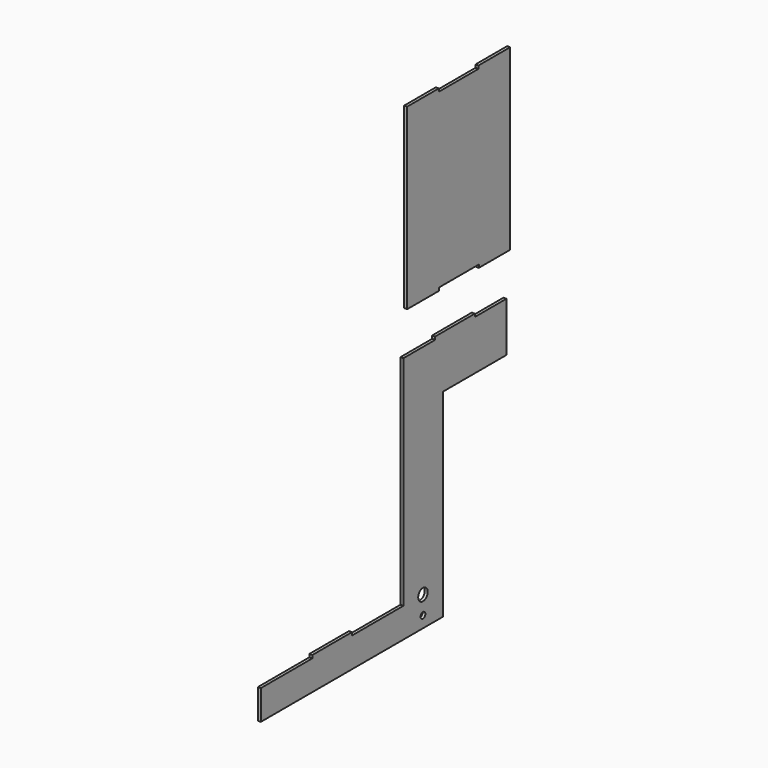
from build123d import *

# Parameters (mm, degrees)
F0_R     = 3
F0_R_2   = 6
F1_DEPTH = 3


with BuildPart() as f1:
    # F0 (on Right) → F1 (new body)
    with BuildSketch(Plane.YZ):
        Polygon((-263.0525815487, 42.160961777), (-298.0525815487, 42.160961777), (-303.0525815487, 42.160961777), (-303.0525815487, 37.160961777), (-303.0525815487, -177.839038223), (-368.0525815487, -177.839038223), (-368.0525815487, -174.839038223), (-418.0525815487, -174.839038223), (-418.0525815487, -177.839038223), (-483.0525815487, -177.839038223), (-483.0525815487, -207.839038223), (-253.0525815487, -207.839038223), (-253.0525815487, -12.839038223), (-253.0525815487, -7.839038223), (-248.0525815487, -7.839038223), (-178.0525815487, -7.839038223), (-173.0525815487, -7.839038223), (-173.0525815487, -2.839038223), (-173.0525815487, 37.160961777), (-173.0525815487, 42.160961777), (-178.0525815487, 42.160961777), (-213.0525815487, 42.160961777), (-213.0525815487, 45.160961777), (-263.0525815487, 45.160961777), align=None)
        with Locations((-278.4440219402, -196.3103711605)):
            Circle(F0_R, mode=Mode.SUBTRACT)
        with Locations((-278.4440219402, -177.839038223)):
            Circle(F0_R_2, mode=Mode.SUBTRACT)
    extrude(amount=-F1_DEPTH)


with BuildPart() as f1b:
    # F0 (on Right) → F1, piece 2 (new body)
    with BuildSketch(Plane.YZ):
        Polygon((-298.3582913876, 263.7473198771), (-298.3582913876, 83.7473198771), (-258.0111324787, 83.7473198771), (-258.0111324787, 86.7473198771), (-208.0111324787, 86.7473198771), (-208.0111324787, 83.7473198771), (-168.3582913876, 83.7473198771), (-168.3582913876, 263.7473198771), (-208.3582913876, 263.7473198771), (-208.3582913876, 260.7473198771), (-258.3582913876, 260.7473198771), (-258.3582913876, 263.7473198771), align=None)
    extrude(amount=-F1_DEPTH)


solid = Compound([f1.part, f1b.part])
